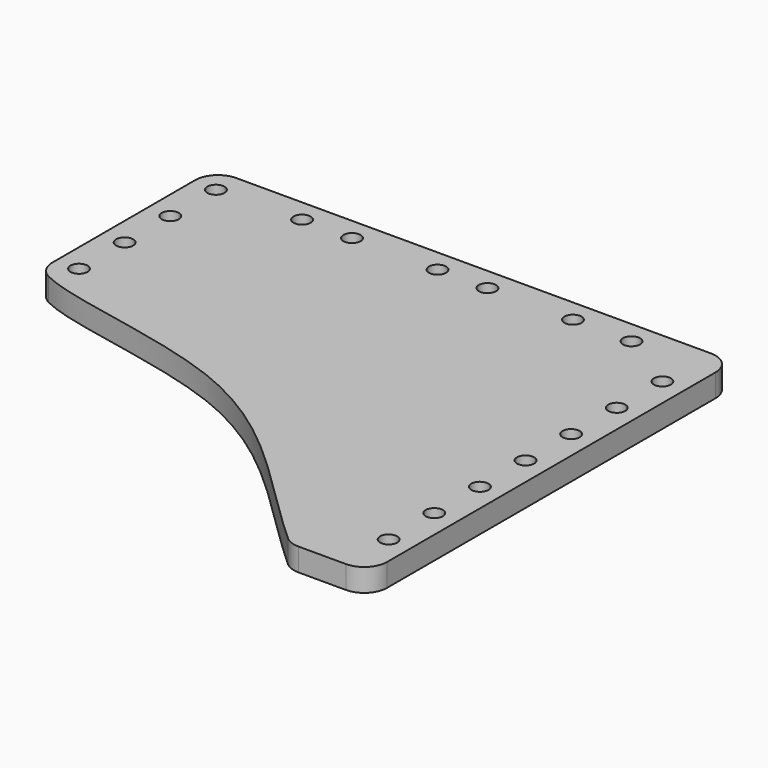
from build123d import *

# Parameters (mm, degrees)
F1_DEPTH = 5.08
F2_R     = 5.08
F2_R_2   = 5.07999
F3_R     = 1.905
F4_DEPTH = 5.0810001


# Not quite as in the source:
# - a fillet or chamfer is up to 0.001 mm smaller than in the source, because OpenCascade refuses the exact size


with BuildPart() as f1:
    # F0 (on Top) → F1 (new body)
    with BuildSketch(Plane.XY):
        with BuildLine():
            Line((-70.1164795637, 40.014226675), (-70.1164795637, -7.2926129862))
            add(Edge.make_bspline(
                [(-70.1164795637, -7.2926129862), (-65.04872861, -13.3058879533), (-12.1612328693, -14.8475963345), (11.7038576667, -47.1047081721), (28.178319335, -61.585773325)],
                knots=[0, 0, 0, 0, 0.4703732395, 1, 1, 1, 1], degree=3))
            Line((28.178319335, -61.585773325), (45.7710204363, -61.585773325))
            Line((45.7710204363, -61.585773325), (45.7710204363, 40.014226675))
            Line((45.7710204363, 40.014226675), (-70.1164795637, 40.014226675))
        make_face()
    extrude(amount=F1_DEPTH)

    # F2 (call 1 of 5: OpenCascade refuses the feature's edges together)
    f2_edges = [f1.edges().sort_by_distance(p)[0] for p in [
        (-70.11648, 40.014227, 2.54),
    ]]
    fillet(f2_edges, radius=F2_R)

    # F2#2 (call 2 of 5)
    f2_2_edges = [f1.edges().sort_by_distance(p)[0] for p in [
        (45.77102, 40.014227, 2.54),
    ]]
    fillet(f2_2_edges, radius=F2_R)

    # F2#4 (call 3 of 5)
    f2_4_edges = [f1.edges().sort_by_distance(p)[0] for p in [
        (28.178319, -61.585773, 2.54),
    ]]
    fillet(f2_4_edges, radius=F2_R)

    # F2#5 (call 4 of 5)
    f2_5_edges = [f1.edges().sort_by_distance(p)[0] for p in [
        (45.77102, -61.585773, 2.54),
    ]]
    fillet(f2_5_edges, radius=F2_R)

    # F2#3 (call 5 of 5) (radius 5.08 in the source; OpenCascade refuses exactly that, so slightly less here)
    f2_3_edges = [f1.edges().sort_by_distance(p)[0] for p in [
        (-70.11648, -7.292613, 2.54),
    ]]
    fillet(f2_3_edges, radius=F2_R_2)

    # F3 (on face) → F4 (cut, through all)
    with BuildSketch(Plane.XY.offset(5.08)):
        with Locations((-46.3039795637, 34.934226675)):
            Circle(F3_R)
        with Locations((-35.1914795637, 34.934226675)):
            Circle(F3_R)
        with Locations((-16.1414795637, 34.934226675)):
            Circle(F3_R)
        with Locations((-5.0289795637, 34.934226675)):
            Circle(F3_R)
        with Locations((14.0210204363, 34.934226675)):
            Circle(F3_R)
        with Locations((-65.0364795637, 34.3525031737)):
            Circle(F3_R)
        with Locations((-65.0364795637, 21.6525031737)):
            Circle(F3_R)
        with Locations((-65.0364795637, 8.9525031737)):
            Circle(F3_R)
        with Locations((-65.0364795637, -3.7474968263)):
            Circle(F3_R)
        with Locations((27.0512204363, 34.934226675)):
            Circle(F3_R)
        with Locations((40.6910204363, 26.4864852548)):
            Circle(F3_R)
        with Locations((40.6910204363, 13.7864852548)):
            Circle(F3_R)
        with Locations((40.6910204363, 1.0864852548)):
            Circle(F3_R)
        with Locations((40.6910204363, -11.6135147452)):
            Circle(F3_R)
        with Locations((40.6910204363, -24.3135147452)):
            Circle(F3_R)
        with Locations((40.6910204363, -37.0135147452)):
            Circle(F3_R)
        with Locations((40.6910204363, -49.7135147452)):
            Circle(F3_R)
    extrude(amount=-F4_DEPTH, mode=Mode.SUBTRACT)


solid = f1.part
